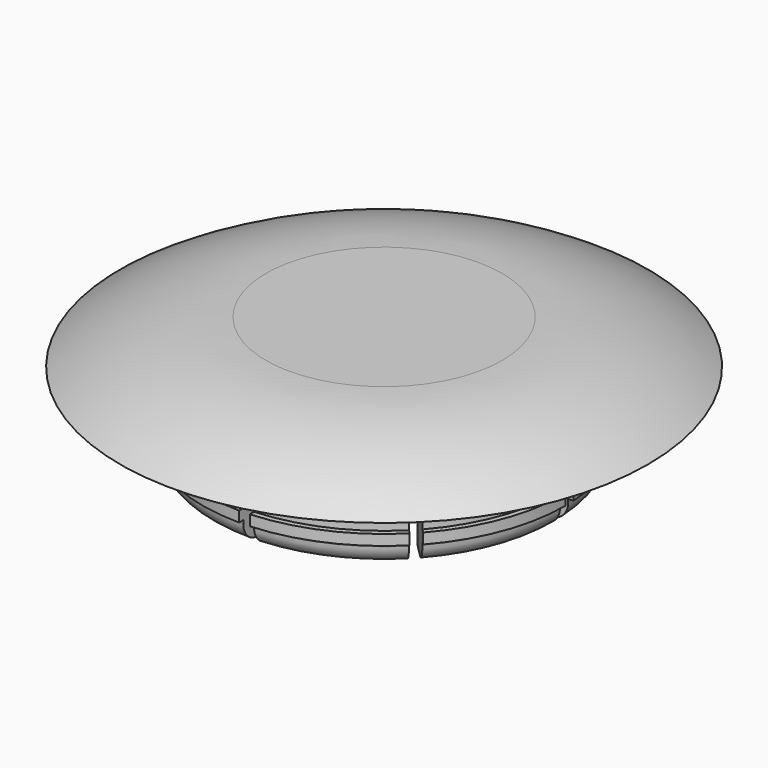
from build123d import *

# Parameters (mm, degrees)
F0_R      = 7.5
F0_R_2    = 5
F0_R_3    = 4.25
F1_DEPTH  = 1.25
F3_DEPTH  = 0.3
F4_R      = 5.15
F5_DEPTH  = 0.3
F6_R      = 5
F7_DEPTH  = 0.3
F8_R      = 5.15
F9_DEPTH  = 0.3
F10_R     = 5
F11_DEPTH = 0.3
F12_R     = 5.15
F13_DEPTH = 0.3
F14_R     = 5
F15_DEPTH = 0.6
F16_R     = 0.5
F18_DEPTH = 2.25


# Not quite as in the source:
# - a fillet or chamfer that OpenCascade refuses, or shapes differently, is made with other operations: its cross-section is extruded or revolved along the edge and cut away or added


with BuildPart() as f1:
    # F0 (on Top) → F1 (new body)
    with BuildSketch(Plane.XY):
        Circle(F0_R)
        Circle(F0_R_2, mode=Mode.SUBTRACT)
        Circle(F0_R_2)
        Circle(F0_R_3, mode=Mode.SUBTRACT)
        Circle(F0_R_3)
    extrude(amount=F1_DEPTH)

    # F2: fillet of radius 7.5 on 1 edges, made by hand

    # F2_s1 → F2_t2 (revolve, cut)
    with BuildSketch(Plane.XZ):
        with BuildLine():
            ThreePointArc((7.5, 0), (5.5192825215, 0.9307033082), (3.354219012, 1.25))
            Line((3.354219012, 1.25), (7.5, 1.25))
            Line((7.5, 1.25), (7.5, 0))
        make_face()
    revolve(axis=Axis((0, 0, 1.25), (0, 0, 1)), mode=Mode.SUBTRACT)

    # F0 (on Top) → F3 (join)
    with BuildSketch(Plane.XY):
        Circle(F0_R_2)
        Circle(F0_R_3, mode=Mode.SUBTRACT)
    extrude(amount=-F3_DEPTH)

    # F4 (on face) → F5 (join)
    with BuildSketch(Plane(origin=(0, 0, -0.3), x_dir=(1, 0, 0), z_dir=(0, 0, -1))):
        Circle(F4_R)
    extrude(amount=F5_DEPTH)

    # F6 (on face) → F7 (join)
    with BuildSketch(Plane(origin=(0, 0, -0.6), x_dir=(1, 0, 0), z_dir=(0, 0, -1))):
        Circle(F6_R)
    extrude(amount=F7_DEPTH)

    # F8 (on face) → F9 (join)
    with BuildSketch(Plane(origin=(0, 0, -0.9), x_dir=(1, 0, 0), z_dir=(0, 0, -1))):
        Circle(F8_R)
    extrude(amount=F9_DEPTH)

    # F10 (on face) → F11 (join)
    with BuildSketch(Plane(origin=(0, 0, -1.2), x_dir=(1, 0, 0), z_dir=(0, 0, -1))):
        Circle(F10_R)
    extrude(amount=F11_DEPTH)

    # F12 (on face) → F13 (join)
    with BuildSketch(Plane(origin=(0, 0, -1.5), x_dir=(1, 0, 0), z_dir=(0, 0, -1))):
        Circle(F12_R)
    extrude(amount=F13_DEPTH)

    # F14 (on face) → F15 (join)
    with BuildSketch(Plane(origin=(0, 0, -1.8), x_dir=(1, 0, 0), z_dir=(0, 0, -1))):
        Circle(F14_R)
    extrude(amount=F15_DEPTH)

    # F16
    f16_edges = [f1.edges().sort_by_distance(p)[0] for p in [
        (-5, 0, -2.4),
    ]]
    fillet(f16_edges, radius=F16_R)

    # F17 (on face) → F18 (cut)
    with BuildSketch(Plane(origin=(0, 0, -2.4), x_dir=(1, 0, 0), z_dir=(0, 0, -1))):
        with BuildLine():
            Line((0.4242640687, 0), (4, 0))
            ThreePointArc((4, 0), (3.7503581135, 1.3909759239), (3.0325929896, 2.6083289209))
            Line((3.0325929896, 2.6083289209), (0.4242640687, 0))
        make_face()
        with BuildLine():
            Line((4.5, 0), (4, 0))
            ThreePointArc((4, 0), (3.9971825415, -0.1501057292), (3.988734135, -0.3))
            Line((3.988734135, -0.3), (4.4899888641, -0.3))
            ThreePointArc((4.4899888641, -0.3), (4.4974965197, -0.1500834958), (4.5, 0))
        make_face()
        with BuildLine():
            ThreePointArc((3.988734135, -0.3), (3.9971825415, -0.1501057292), (4, 0))
            Line((4, 0), (0.4242640687, 0))
            Line((0.4242640687, 0), (0.2121320344, -0.2121320344))
            Line((0.2121320344, -0.2121320344), (0.3, -0.3))
            Line((0.3, -0.3), (3.988734135, -0.3))
        make_face()
        with BuildLine():
            Line((0.4242640687, 0), (3.0325929896, 2.6083289209))
            ThreePointArc((3.0325929896, 2.6083289209), (2.9325756597, 2.7202941017), (2.8284271247, 2.8284271247))
            Line((2.8284271247, 2.8284271247), (0.3, 0.3))
            Line((0.3, 0.3), (0.3, 0))
            Line((0.3, 0), (0.4242640687, 0))
        make_face()
        with BuildLine():
            ThreePointArc((2.8284271247, 2.8284271247), (2.9325756597, 2.7202941017), (3.0325929896, 2.6083289209))
            Line((3.0325929896, 2.6083289209), (3.3870336076, 2.9627695389))
            ThreePointArc((3.3870336076, 2.9627695389), (3.286335345, 3.0740852298), (3.1819805153, 3.1819805153))
            Line((3.1819805153, 3.1819805153), (2.8284271247, 2.8284271247))
        make_face()
        with BuildLine():
            ThreePointArc((2.8284271247, -2.8284271247), (3.6354721621, -1.6683351457), (3.988734135, -0.3))
            Line((3.988734135, -0.3), (0.3, -0.3))
            Line((0.3, -0.3), (2.8284271247, -2.8284271247))
        make_face()
        with BuildLine():
            Line((6, 0), (4.5, 0))
            ThreePointArc((4.5, 0), (4.4974965197, -0.1500834958), (4.4899888641, -0.3))
            Line((4.4899888641, -0.3), (6, -0.3))
            Line((6, -0.3), (6, 0))
        make_face()
        Polygon((0.2121320344, -0.2121320344), (0.4242640687, 0), (0.3, 0), (0, 0), align=None)
        with BuildLine():
            Line((0.3, 0.3), (2.8284271247, 2.8284271247))
            ThreePointArc((2.8284271247, 2.8284271247), (1.6683351457, 3.6354721621), (0.3, 3.988734135))
            Line((0.3, 3.988734135), (0.3, 0.3))
        make_face()
        with BuildLine():
            ThreePointArc((3.1819805153, 3.1819805153), (3.286335345, 3.0740852298), (3.3870336076, 2.9627695389))
            Line((3.3870336076, 2.9627695389), (4.4547727215, 4.0305086528))
            Line((4.4547727215, 4.0305086528), (4.2426406871, 4.2426406871))
            Line((4.2426406871, 4.2426406871), (3.1819805153, 3.1819805153))
        make_face()
        with BuildLine():
            Line((3.1819805153, -3.1819805153), (2.8284271247, -2.8284271247))
            ThreePointArc((2.8284271247, -2.8284271247), (2.7202941017, -2.9325756597), (2.6083289209, -3.0325929896))
            Line((2.6083289209, -3.0325929896), (2.9627695389, -3.3870336076))
            ThreePointArc((2.9627695389, -3.3870336076), (3.0740852298, -3.286335345), (3.1819805153, -3.1819805153))
        make_face()
        with BuildLine():
            ThreePointArc((2.6083289209, -3.0325929896), (2.7202941017, -2.9325756597), (2.8284271247, -2.8284271247))
            Line((2.8284271247, -2.8284271247), (0.3, -0.3))
            Line((0.3, -0.3), (0, -0.3))
            Line((0, -0.3), (0, -0.4242640687))
            Line((0, -0.4242640687), (2.6083289209, -3.0325929896))
        make_face()
        Polygon((0, -0.3), (0.3, -0.3), (0.2121320344, -0.2121320344), (0, 0), align=None)
        Polygon((0, 0), (0.3, 0), (0.3, 0.3), (0.2121320344, 0.2121320344), align=None)
        with BuildLine():
            Line((0.3, 0.3), (0.3, 3.988734135))
            ThreePointArc((0.3, 3.988734135), (0.1501057292, 3.9971825415), (0, 4))
            Line((0, 4), (0, 0.4242640687))
            Line((0, 0.4242640687), (0.2121320344, 0.2121320344))
            Line((0.2121320344, 0.2121320344), (0.3, 0.3))
        make_face()
        with BuildLine():
            ThreePointArc((0, 4), (0.1501057292, 3.9971825415), (0.3, 3.988734135))
            Line((0.3, 3.988734135), (0.3, 4.4899888641))
            ThreePointArc((0.3, 4.4899888641), (0.1500834958, 4.4974965197), (0, 4.5))
            Line((0, 4.5), (0, 4))
        make_face()
        with BuildLine():
            ThreePointArc((0, -4), (1.3909759239, -3.7503581135), (2.6083289209, -3.0325929896))
            Line((2.6083289209, -3.0325929896), (0, -0.4242640687))
            Line((0, -0.4242640687), (0, -4))
        make_face()
        with BuildLine():
            Line((4.2426406871, -4.2426406871), (3.1819805153, -3.1819805153))
            ThreePointArc((3.1819805153, -3.1819805153), (3.0740852298, -3.286335345), (2.9627695389, -3.3870336076))
            Line((2.9627695389, -3.3870336076), (4.0305086528, -4.4547727215))
            Line((4.0305086528, -4.4547727215), (4.2426406871, -4.2426406871))
        make_face()
        Polygon((0, -0.4242640687), (0, -0.3), (0, 0), (-0.2121320344, -0.2121320344), align=None)
        Polygon((-0.2121320344, 0.2121320344), (0, 0), (0, 0.3), (-0.3, 0.3), align=None)
        Polygon((-0.3, 0), (0, 0), (-0.2121320344, 0.2121320344), (-0.4242640687, 0), align=None)
        Polygon((-0.2121320344, -0.2121320344), (0, 0), (-0.3, 0), (-0.3, -0.3), align=None)
        Polygon((0, 0.3), (0, 0), (0.2121320344, 0.2121320344), (0, 0.4242640687), align=None)
        with BuildLine():
            Line((0, 0.4242640687), (0, 4))
            ThreePointArc((0, 4), (-1.3909759239, 3.7503581135), (-2.6083289209, 3.0325929896))
            Line((-2.6083289209, 3.0325929896), (0, 0.4242640687))
        make_face()
        with BuildLine():
            ThreePointArc((0, 4.5), (0.1500834958, 4.4974965197), (0.3, 4.4899888641))
            Line((0.3, 4.4899888641), (0.3, 6))
            Line((0.3, 6), (0, 6))
            Line((0, 6), (0, 4.5))
        make_face()
        with BuildLine():
            Line((0, -4.5), (0, -4))
            ThreePointArc((0, -4), (-0.1501057292, -3.9971825415), (-0.3, -3.988734135))
            Line((-0.3, -3.988734135), (-0.3, -4.4899888641))
            ThreePointArc((-0.3, -4.4899888641), (-0.1500834958, -4.4974965197), (0, -4.5))
        make_face()
        with BuildLine():
            ThreePointArc((-0.3, -3.988734135), (-0.1501057292, -3.9971825415), (0, -4))
            Line((0, -4), (0, -0.4242640687))
            Line((0, -0.4242640687), (-0.2121320344, -0.2121320344))
            Line((-0.2121320344, -0.2121320344), (-0.3, -0.3))
            Line((-0.3, -0.3), (-0.3, -3.988734135))
        make_face()
        with BuildLine():
            Line((-0.3, 0.3), (0, 0.3))
            Line((0, 0.3), (0, 0.4242640687))
            Line((0, 0.4242640687), (-2.6083289209, 3.0325929896))
            ThreePointArc((-2.6083289209, 3.0325929896), (-2.7202941017, 2.9325756597), (-2.8284271247, 2.8284271247))
            Line((-2.8284271247, 2.8284271247), (-0.3, 0.3))
        make_face()
        with BuildLine():
            Line((-0.4242640687, 0), (-0.2121320344, 0.2121320344))
            Line((-0.2121320344, 0.2121320344), (-0.3, 0.3))
            Line((-0.3, 0.3), (-3.988734135, 0.3))
            ThreePointArc((-3.988734135, 0.3), (-3.9971825415, 0.1501057292), (-4, 0))
            Line((-4, 0), (-0.4242640687, 0))
        make_face()
        with BuildLine():
            Line((-0.3, -0.3), (-0.3, 0))
            Line((-0.3, 0), (-0.4242640687, 0))
            Line((-0.4242640687, 0), (-3.0325929896, -2.6083289209))
            ThreePointArc((-3.0325929896, -2.6083289209), (-2.9325756597, -2.7202941017), (-2.8284271247, -2.8284271247))
            Line((-2.8284271247, -2.8284271247), (-0.3, -0.3))
        make_face()
        with BuildLine():
            ThreePointArc((-2.8284271247, 2.8284271247), (-2.7202941017, 2.9325756597), (-2.6083289209, 3.0325929896))
            Line((-2.6083289209, 3.0325929896), (-2.9627695389, 3.3870336076))
            ThreePointArc((-2.9627695389, 3.3870336076), (-3.0740852298, 3.286335345), (-3.1819805153, 3.1819805153))
            Line((-3.1819805153, 3.1819805153), (-2.8284271247, 2.8284271247))
        make_face()
        with BuildLine():
            ThreePointArc((-2.8284271247, -2.8284271247), (-1.6683351457, -3.6354721621), (-0.3, -3.988734135))
            Line((-0.3, -3.988734135), (-0.3, -0.3))
            Line((-0.3, -0.3), (-2.8284271247, -2.8284271247))
        make_face()
        with BuildLine():
            Line((0, -6), (0, -4.5))
            ThreePointArc((0, -4.5), (-0.1500834958, -4.4974965197), (-0.3, -4.4899888641))
            Line((-0.3, -4.4899888641), (-0.3, -6))
            Line((-0.3, -6), (0, -6))
        make_face()
        with BuildLine():
            Line((-3.988734135, 0.3), (-0.3, 0.3))
            Line((-0.3, 0.3), (-2.8284271247, 2.8284271247))
            ThreePointArc((-2.8284271247, 2.8284271247), (-3.6354721621, 1.6683351457), (-3.988734135, 0.3))
        make_face()
        with BuildLine():
            Line((-3.0325929896, -2.6083289209), (-0.4242640687, 0))
            Line((-0.4242640687, 0), (-4, 0))
            ThreePointArc((-4, 0), (-3.7503581135, -1.3909759239), (-3.0325929896, -2.6083289209))
        make_face()
        with BuildLine():
            ThreePointArc((-3.1819805153, 3.1819805153), (-3.0740852298, 3.286335345), (-2.9627695389, 3.3870336076))
            Line((-2.9627695389, 3.3870336076), (-4.0305086528, 4.4547727215))
            Line((-4.0305086528, 4.4547727215), (-4.2426406871, 4.2426406871))
            Line((-4.2426406871, 4.2426406871), (-3.1819805153, 3.1819805153))
        make_face()
        with BuildLine():
            Line((-3.1819805153, -3.1819805153), (-2.8284271247, -2.8284271247))
            ThreePointArc((-2.8284271247, -2.8284271247), (-2.9325756597, -2.7202941017), (-3.0325929896, -2.6083289209))
            Line((-3.0325929896, -2.6083289209), (-3.3870336076, -2.9627695389))
            ThreePointArc((-3.3870336076, -2.9627695389), (-3.286335345, -3.0740852298), (-3.1819805153, -3.1819805153))
        make_face()
        with BuildLine():
            ThreePointArc((-4, 0), (-3.9971825415, 0.1501057292), (-3.988734135, 0.3))
            Line((-3.988734135, 0.3), (-4.4899888641, 0.3))
            ThreePointArc((-4.4899888641, 0.3), (-4.4974965197, 0.1500834958), (-4.5, 0))
            Line((-4.5, 0), (-4, 0))
        make_face()
        with BuildLine():
            Line((-4.2426406871, -4.2426406871), (-3.1819805153, -3.1819805153))
            ThreePointArc((-3.1819805153, -3.1819805153), (-3.286335345, -3.0740852298), (-3.3870336076, -2.9627695389))
            Line((-3.3870336076, -2.9627695389), (-4.4547727215, -4.0305086528))
            Line((-4.4547727215, -4.0305086528), (-4.2426406871, -4.2426406871))
        make_face()
        with BuildLine():
            ThreePointArc((-4.5, 0), (-4.4974965197, 0.1500834958), (-4.4899888641, 0.3))
            Line((-4.4899888641, 0.3), (-6, 0.3))
            Line((-6, 0.3), (-6, 0))
            Line((-6, 0), (-4.5, 0))
        make_face()
    extrude(amount=-F18_DEPTH, mode=Mode.SUBTRACT)


solid = f1.part
